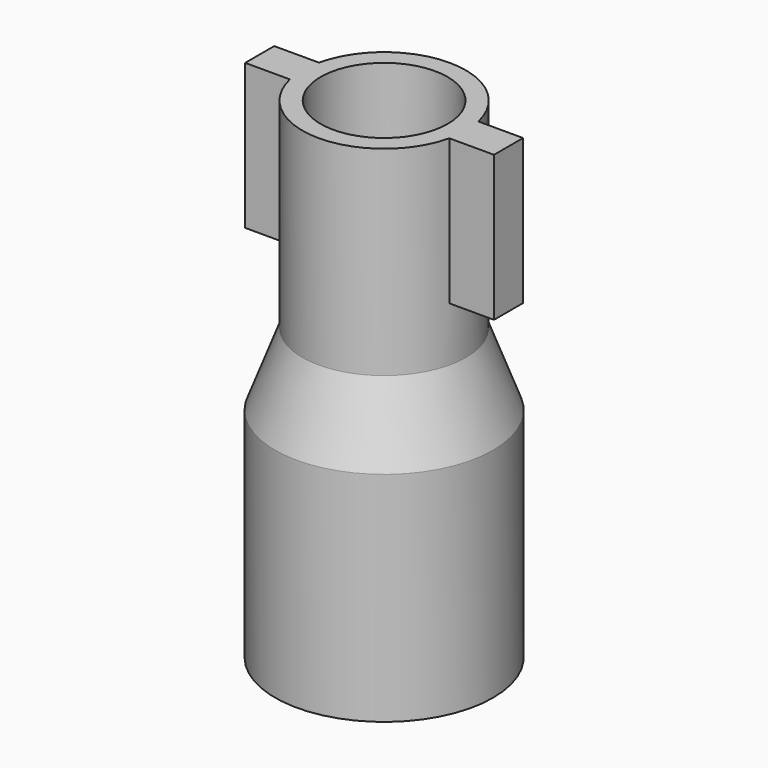
from build123d import *

# Parameters (mm, degrees)
F0_R     = 4.5
F0_R_2   = 3.5
F1_DEPTH = 11
F2_W     = 3.2331479252
F2_H     = 2
F3_DEPTH = 8
F4_R     = 6
F5_DEPTH = 16
F6_SIZE2 = 1.49999
F6_SIZE  = 3.99999
F8_DEPTH = 10


# Not quite as in the source:
# - a fillet or chamfer is up to 0.001 mm smaller than in the source, because OpenCascade refuses the exact size


with BuildPart() as f1:
    # F0 (on Top) → F1 (new body)
    with BuildSketch(Plane.XY):
        Circle(F0_R)
        Circle(F0_R_2, mode=Mode.SUBTRACT)
    extrude(amount=F1_DEPTH)

    # F2 (on face) → F3 (join)
    with BuildSketch(Plane.XY.offset(11)):
        with Locations((-5.2334260374, 0)):
            Rectangle(F2_W, F2_H)
        with Locations((5.2334260374, 0)):
            Rectangle(F2_W, F2_H)
    extrude(amount=-F3_DEPTH)

    # F4 (on face) → F5 (join)
    with BuildSketch(Plane(origin=(0, 0, 0), x_dir=(1, 0, 0), z_dir=(0, 0, -1))):
        Circle(F4_R)
    extrude(amount=F5_DEPTH)

    # F6 (size 4 and 1.5 in the source; OpenCascade refuses exactly that, so slightly less here)
    f6_edges = [f1.edges().sort_by_distance(p)[0] for p in [
        (-6, 0, 0),
    ]]
    f6_side = f1.faces().sort_by_distance((-6, 0, -8))[0]
    chamfer(f6_edges, length=F6_SIZE, length2=F6_SIZE2, reference=f6_side)

    # F7 (on face) → F8 (cut)
    with BuildSketch(Plane(origin=(0, 0, -16), x_dir=(1, 0, 0), z_dir=(0, 0, -1))):
        Polygon((-1.5, 1.5), (-4, 1.5), (-4, -1.5), (-1.5, -1.5), (-1.5, -4), (1.5, -4), (1.5, -1.5), (4, -1.5), (4, 1.5), (1.5, 1.5), (1.5, 4), (-1.5, 4), align=None)
    extrude(amount=-F8_DEPTH, mode=Mode.SUBTRACT)


solid = f1.part
